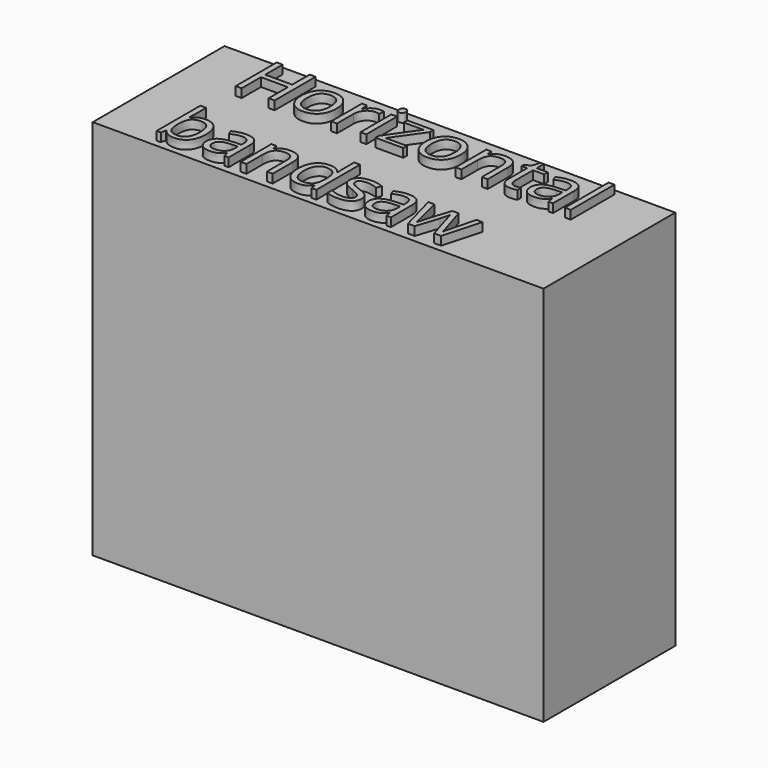
from build123d import *

# Parameters (mm, degrees)
F0_W         = 1320.8
F0_H         = 482.6
F1_DEPTH     = 1117.6
F2_TEXT_SIZE = 210.365577483
F3_DEPTH     = 25.4


# Not quite as in the source:
# - Text() gives the source's letters only with a copy of the font that has no kerning and outlines rounded to 1/6400 em; it was checked with that copy


with BuildPart() as f1:
    # F0 (on Top) → F1 (new body)
    with BuildSketch(Plane.XY):
        with Locations((-1.2626160169, 0)):
            Rectangle(F0_W, F0_H)
    extrude(amount=F1_DEPTH)

    # F2 (on face) → F3 (join)
    with BuildSketch(Plane.XY.offset(1117.6)):
        with Locations((-508, 64.4367842122)):
            Text('Horizontal', F2_TEXT_SIZE, font='Open Sans', text_align=(TextAlign.LEFT, TextAlign.BOTTOM))
        with Locations((-508, -221.6604011647)):
            Text('bandsaw', F2_TEXT_SIZE, font='Open Sans', text_align=(TextAlign.LEFT, TextAlign.BOTTOM))
    extrude(amount=F3_DEPTH)


solid = f1.part
